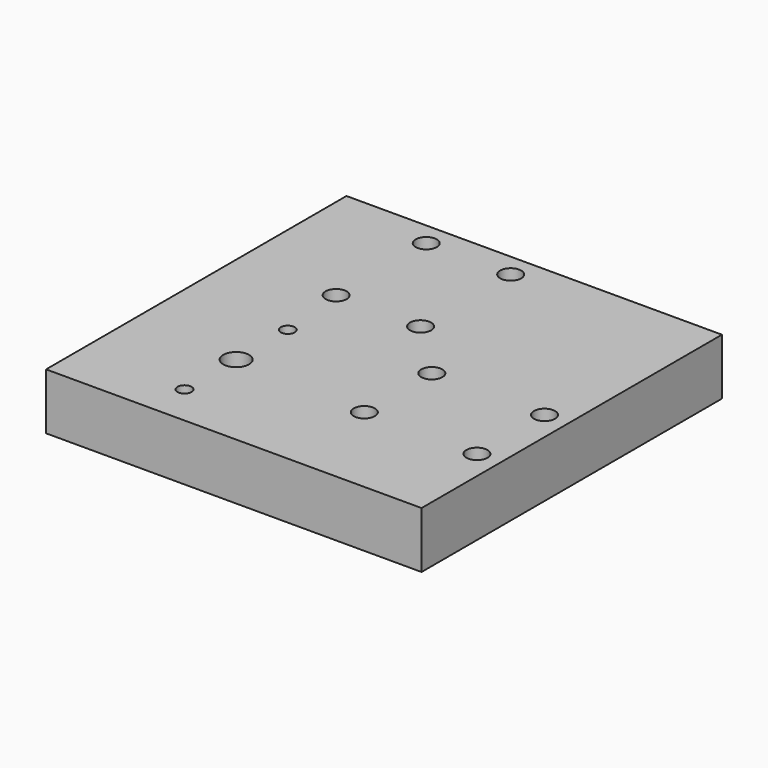
from build123d import *

# Parameters (mm, degrees)
F0_W     = 80
F0_H     = 80
F0_R     = 1.5
F0_R_2   = 2.75
F0_R_3   = 2.25
F1_DEPTH = 12


with BuildPart() as f1:
    # F0 (on Top) → F1 (new body)
    with BuildSketch(Plane.XY):
        with Locations((40, 40)):
            Rectangle(F0_W, F0_H)
        with Locations((22.5, 8.75)):
            Circle(F0_R, mode=Mode.SUBTRACT)
        with Locations((22.5, 22.5)):
            Circle(F0_R_2, mode=Mode.SUBTRACT)
        with Locations((22.5, 36.25)):
            Circle(F0_R, mode=Mode.SUBTRACT)
        with Locations((51, 21)):
            Circle(F0_R_3, mode=Mode.SUBTRACT)
        with Locations((51, 39)):
            Circle(F0_R_3, mode=Mode.SUBTRACT)
        with Locations((75, 21)):
            Circle(F0_R_3, mode=Mode.SUBTRACT)
        with Locations((75, 39)):
            Circle(F0_R_3, mode=Mode.SUBTRACT)
        with Locations((21, 51)):
            Circle(F0_R_3, mode=Mode.SUBTRACT)
        with Locations((39, 51)):
            Circle(F0_R_3, mode=Mode.SUBTRACT)
        with Locations((21, 75)):
            Circle(F0_R_3, mode=Mode.SUBTRACT)
        with Locations((39, 75)):
            Circle(F0_R_3, mode=Mode.SUBTRACT)
    extrude(amount=F1_DEPTH)


solid = f1.part
